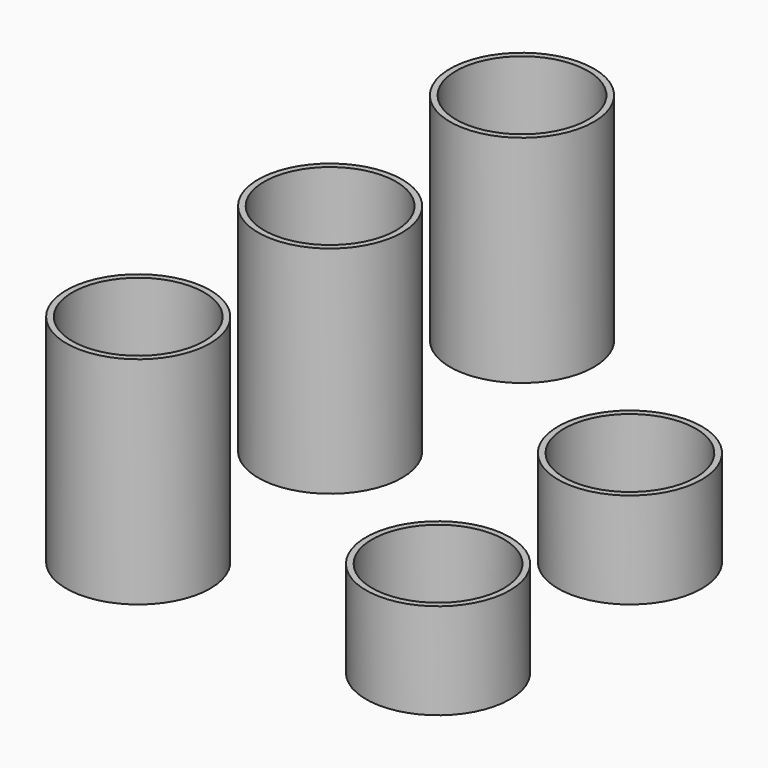
from build123d import *

# Parameters (mm, degrees)
F0_R     = 6
F0_R_2   = 5.5
F1_DEPTH = 18
F2_DEPTH = 8
F0_R_3   = 2.4
F0_R_4   = 1.9
F0_R_5   = 0.75
F3_DEPTH = 1.5


with BuildPart() as f1:
    # F0 (on Top) → F1 (new body)
    with BuildSketch(Plane.XY):
        Circle(F0_R)
        Circle(F0_R_2, mode=Mode.SUBTRACT)
    extrude(amount=F1_DEPTH)


with BuildPart() as f1b:
    # F0 (on Top) → F1, piece 2 (new body)
    with BuildSketch(Plane.XY):
        with Locations((0, 20)):
            Circle(F0_R)
        with Locations((0, 20)):
            Circle(F0_R_2, mode=Mode.SUBTRACT)
    extrude(amount=F1_DEPTH)


with BuildPart() as f1c:
    # F0 (on Top) → F1, piece 3 (new body)
    with BuildSketch(Plane.XY):
        with Locations((0, 40)):
            Circle(F0_R)
        with Locations((0, 40)):
            Circle(F0_R_2, mode=Mode.SUBTRACT)
    extrude(amount=F1_DEPTH)


with BuildPart() as f2:
    # F0 (on Top) → F2 (new body)
    with BuildSketch(Plane.XY):
        with Locations((25, 0)):
            Circle(F0_R)
        with Locations((25, 0)):
            Circle(F0_R_2, mode=Mode.SUBTRACT)
    extrude(amount=F2_DEPTH)

    # F0 (on Top) → F3 (join)
    with BuildSketch(Plane.XY):
        with Locations((25, 0)):
            Circle(F0_R_2)
        with Locations((25, 0)):
            Circle(F0_R_3, mode=Mode.SUBTRACT)
        with Locations((25, 0)):
            Circle(F0_R_3)
        with Locations((25, 0)):
            Circle(F0_R_4, mode=Mode.SUBTRACT)
        with Locations((25, 0)):
            Circle(F0_R_4)
        with Locations((25, 0)):
            Circle(F0_R_5, mode=Mode.SUBTRACT)
    extrude(amount=F3_DEPTH)


with BuildPart() as f2b:
    # F0 (on Top) → F2, piece 2 (new body)
    with BuildSketch(Plane.XY):
        with Locations((25, 20)):
            Circle(F0_R)
        with Locations((25, 20)):
            Circle(F0_R_2, mode=Mode.SUBTRACT)
    extrude(amount=F2_DEPTH)


with BuildPart() as f3:
    # F0 (on Top) → F3, piece 2 (new body)
    with BuildSketch(Plane.XY):
        with Locations((25, 20)):
            Circle(F0_R_2)
        with Locations((25, 20)):
            Circle(F0_R_3, mode=Mode.SUBTRACT)
        with Locations((25, 20)):
            Circle(F0_R_3)
        with Locations((25, 20)):
            Circle(F0_R_4, mode=Mode.SUBTRACT)
        with Locations((25, 20)):
            Circle(F0_R_4)
        with Locations((25, 20)):
            Circle(F0_R_5, mode=Mode.SUBTRACT)
    extrude(amount=F3_DEPTH)


solid = Compound([f1.part, f1b.part, f1c.part, f2.part, f2b.part, f3.part])
